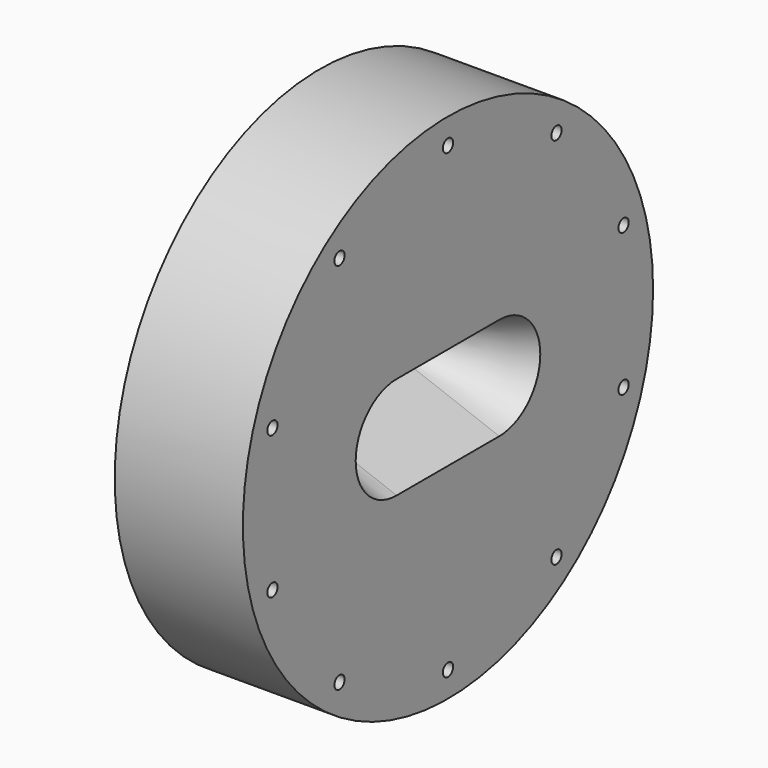
from build123d import *

# Parameters (mm, degrees)
F0_R            = 12.7
F1_DEPTH        = 3.175
F2_R            = 0.3175
F4_DEPTH        = 6.351
F4_COPIES_COUNT = 10
F7_DEPTH        = 0.254


# Not quite as in the source:
# - a pattern or mirror of a feature is missing from the dataset's text; its kind, count and spacing are read off the source's solid


with BuildPart() as f1:
    # F0 (on Right) → F1 (new body, symmetric)
    with BuildSketch(Plane.YZ):
        Circle(F0_R)
    extrude(amount=F1_DEPTH, both=True)

    # F2 (on face) → F4 (cut, through all)
    with BuildSketch(Plane(origin=(-3.175, 0, 0), x_dir=(0, -1, 0), z_dir=(-1, 0, 0))):
        with Locations((0, 11.43)):
            Circle(F2_R)
    f4 = extrude(amount=-F4_DEPTH, mode=Mode.SUBTRACT)

    # F4_copies: F4 ×10 about axis
    f4_copies_axis = Axis((0, 0, 0), (1, 0, 0))
    for i in range(1, F4_COPIES_COUNT):
        add(f4.rotate(f4_copies_axis, i * 360 / F4_COPIES_COUNT), mode=Mode.SUBTRACT)

    # F5 (on face) → F7 (cut)
    with BuildSketch(Plane(origin=(-3.175, 0, 0), x_dir=(0, -1, 0), z_dir=(-1, 0, 0))):
        with BuildLine():
            ThreePointArc((-3.175, 0.254), (-3.429, 0), (-3.175, -0.254))
            Line((-3.175, -0.254), (0, -0.254))
            Line((0, -0.254), (3.175, -0.254))
            ThreePointArc((3.175, -0.254), (3.429, 0), (3.175, 0.254))
            Line((3.175, 0.254), (0, 0.254))
            Line((0, 0.254), (-3.175, 0.254))
        make_face()
    extrude(amount=-F7_DEPTH, mode=Mode.SUBTRACT)

    # F6 (on face) → F9 section 0
    with BuildSketch(Plane.YZ.offset(3.175)):
        with BuildLine():
            ThreePointArc((-3.175, 2.54), (-5.715, 0), (-3.175, -2.54))
            Line((-3.175, -2.54), (0, -2.54))
            Line((0, -2.54), (3.175, -2.54))
            ThreePointArc((3.175, -2.54), (5.715, 0), (3.175, 2.54))
            Line((3.175, 2.54), (0, 2.54))
            Line((0, 2.54), (-3.175, 2.54))
        make_face()
    # F8 (on face) → F9 section 1
    with BuildSketch(Plane(origin=(-2.921, 0, 0), x_dir=(0, -1, 0), z_dir=(-1, 0, 0))):
        with BuildLine():
            ThreePointArc((-3.175, 0.254), (-3.429, 0), (-3.175, -0.254))
            Line((-3.175, -0.254), (0, -0.254))
            Line((0, -0.254), (3.175, -0.254))
            ThreePointArc((3.175, -0.254), (3.429, 0), (3.175, 0.254))
            Line((3.175, 0.254), (0, 0.254))
            Line((0, 0.254), (-3.175, 0.254))
        make_face()
    loft(mode=Mode.SUBTRACT)


solid = f1.part
